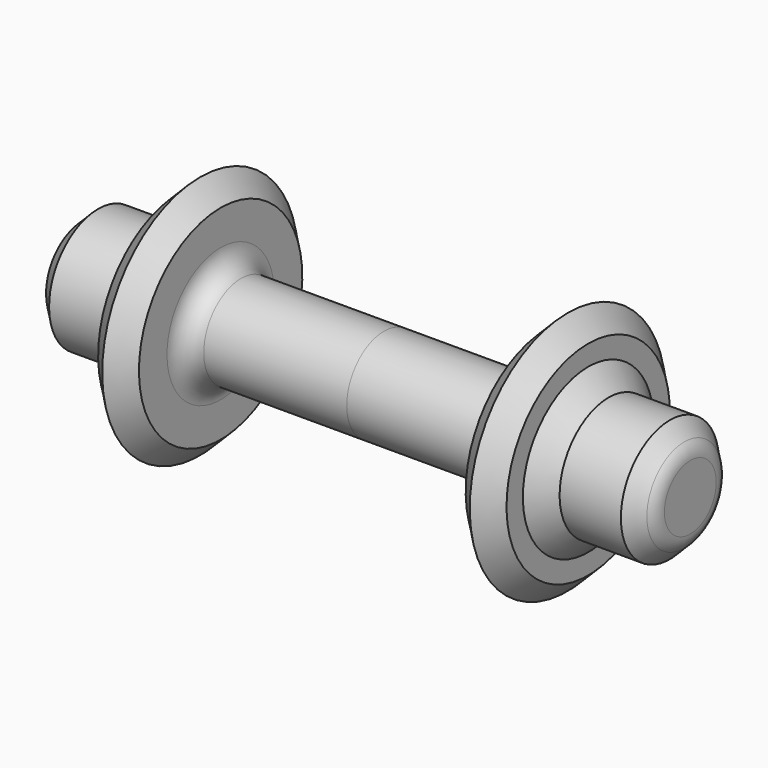
from build123d import *

# Parameters (mm, degrees)
F3_SIZE = 4.99999
F4_R    = 5


# Not quite as in the source:
# - a fillet or chamfer is up to 0.001 mm smaller than in the source, because OpenCascade refuses the exact size


with BuildPart() as f1:
    # F0 (on Front) → F1 (revolve)
    with BuildSketch(Plane.XZ):
        with BuildLine():
            Line((0, 11.4077670069), (0, 0))
            Line((0, 0), (75, 0))
            Line((75, 0), (75, 15))
            Line((75, 15), (50, 15))
            Line((50, 15), (50, 30))
            Line((50, 30), (40, 30))
            Line((40, 30), (40, 16.4077670069))
            ThreePointArc((40, 16.4077670069), (38.5355339059, 12.872233101), (35, 11.4077670069))
            Line((35, 11.4077670069), (0, 11.4077670069))
        make_face()
    revolve(axis=Axis((37.5, 0, 0), (-1, 0, 0)))

    # F2: F1 across face


with BuildPart() as f1_1:
    add(f1.part)
    add(f1.part.mirror(Plane(origin=(0, 0, 0), x_dir=(0, -1, 0), z_dir=(-1, 0, 0))))

    # F3 (size 5 in the source; OpenCascade refuses exactly that, so slightly less here)
    f3_edges = [f1_1.edges().sort_by_distance(p)[0] for p in [
        (-40, 0, -30),
        (-75, 0, -15),
        (-50, 0, -30),
        (40, 0, -30),
        (40, 0, -16.407767),
        (-35, 0, -11.407767),
        (35, 0, -11.407767),
        (75, 0, -15),
        (50, 0, -30),
        (-40, 0, -16.407767),
        (-50, 0, -15),
        (50, 0, -15),
    ]]
    chamfer(f3_edges, length=F3_SIZE)

    # F4
    f4_edges = [f1_1.edges().sort_by_distance(p)[0] for p in [
        (-75, 0, -10.00001),
        (75, 0, -10.00001),
    ]]
    fillet(f4_edges, radius=F4_R)


solid = f1_1.part
